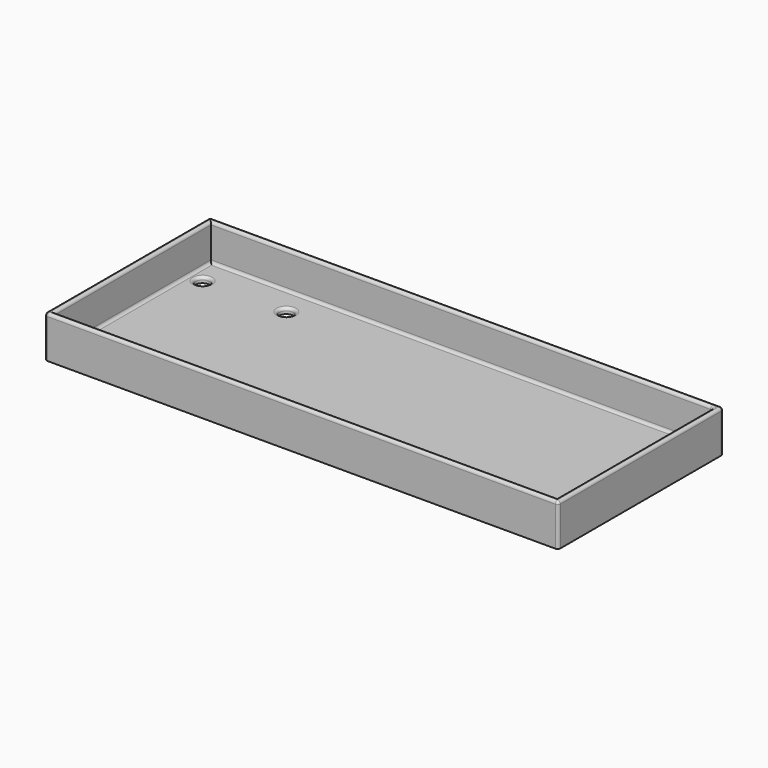
from build123d import *

# Parameters (mm, degrees)
F0_W     = 180
F0_H     = 70
F0_R     = 2.5
F1_DEPTH = 2
F0_W_2   = 184
F0_H_2   = 74
F2_DEPTH = 15
F3_DEPTH = 25
F4_R     = 0.99999


# Not quite as in the source:
# - a fillet or chamfer is up to 0.001 mm smaller than in the source, because OpenCascade refuses the exact size
# - a feature names something its author has since deleted; it is built from what else it names


with BuildPart() as f1:
    # F0 (on Top) → F1 (new body)
    with BuildSketch(Plane.XY):
        Rectangle(F0_W, F0_H)
        with Locations((-85, -25)):
            Circle(F0_R, mode=Mode.SUBTRACT)
        with Locations((-55, -25)):
            Circle(F0_R, mode=Mode.SUBTRACT)
        with Locations((-85, 25)):
            Circle(F0_R, mode=Mode.SUBTRACT)
        with Locations((-55, 25)):
            Circle(F0_R, mode=Mode.SUBTRACT)
        with Locations((85, 0)):
            Circle(F0_R, mode=Mode.SUBTRACT)
    extrude(amount=F1_DEPTH)

    # F0 (on Top) → F2 (join)
    with BuildSketch(Plane.XY):
        Rectangle(F0_W_2, F0_H_2)
        Rectangle(F0_W, F0_H, mode=Mode.SUBTRACT)
    extrude(amount=F2_DEPTH)

    # F0 (on Top) → F3 (cut)
    with BuildSketch(Plane.XY):
        with Locations((-55, -25)):
            Circle(F0_R)
        with Locations((-85, -25)):
            Circle(F0_R)
        with Locations((-85, 25)):
            Circle(F0_R)
        with Locations((-55, 25)):
            Circle(F0_R)
    extrude(amount=-F3_DEPTH, mode=Mode.SUBTRACT)

    # F4 (radius 1 in the source; OpenCascade refuses exactly that, so slightly less here)
    f4_edges = [f1.edges().sort_by_distance(p)[0] for p in [
        (92, 37, 7.5),
        (90, 35, 8.5),
        (0, 37, 15),
        (-92, 0, 15),
        (0, -37, 15),
        (92, 0, 15),
        (0, 35, 15),
        (90, 0, 15),
        (0, -35, 15),
        (-90, 0, 15),
        (92, -37, 7.5),
        (-92, -37, 7.5),
        (-92, 37, 7.5),
        (90, 0, 2),
        (0, 35, 2),
        (-90, 0, 2),
        (0, -35, 2),
        (-87.5, -25, 2),
        (-57.5, -25, 2),
        (-87.5, 25, 2),
        (-57.5, 25, 2),
        (82.5, 0, 2),
    ]]
    fillet(f4_edges, radius=F4_R)


solid = f1.part
